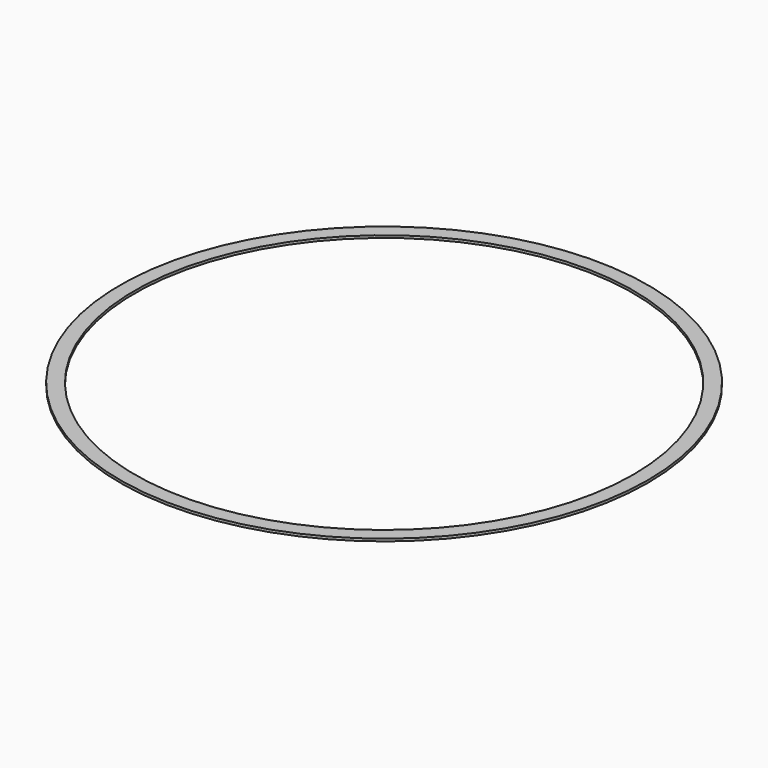
from build123d import *

# Parameters (mm, degrees)
F0_R     = 456.26782
F0_R_2   = 430.86782
F1_DEPTH = 4.2333333333
F2_DEPTH = 4.2333333333


# Not quite as in the source:
# - a length typed as a fraction of an inch, garbled in the dataset ("3 / 203.2 mm" for 3/8 in), is restored


with BuildPart() as f1:
    # F0 (on Top) → F1 (new body)
    with BuildSketch(Plane.XY):
        Circle(F0_R)
        Circle(F0_R_2, mode=Mode.SUBTRACT)
    extrude(amount=F1_DEPTH)


with BuildPart() as f2:
    # F0 (on Top) → F2 (new body)
    with BuildSketch(Plane.XY):
        Circle(F0_R)
        Circle(F0_R_2, mode=Mode.SUBTRACT)
    extrude(amount=F2_DEPTH)


solid = Compound([f1.part, f2.part])
